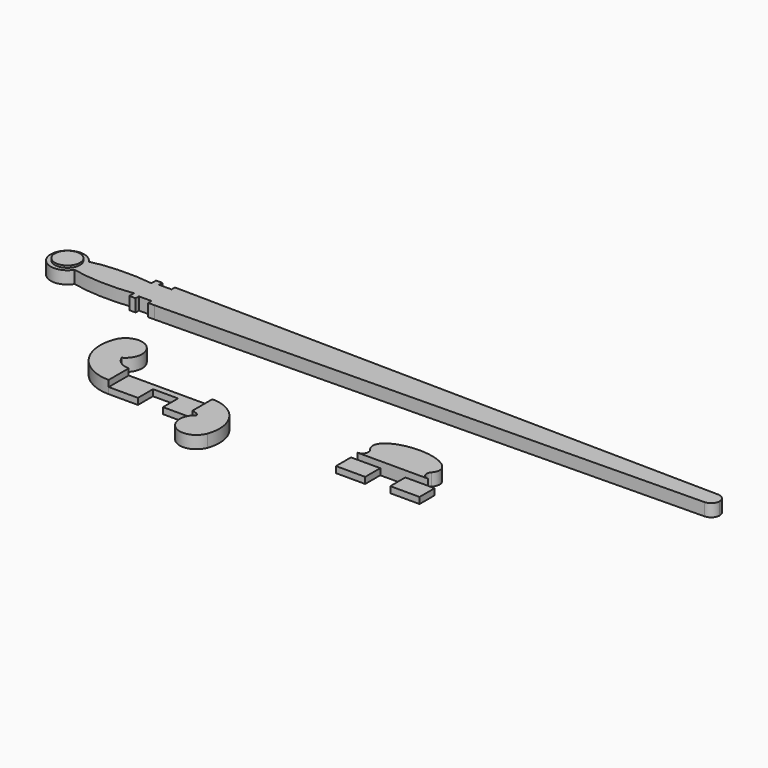
from build123d import *

# Parameters (mm, degrees)
F1_DEPTH      = 15
F0_W          = 35
F0_H          = 7.5
F2_DEPTH      = 7.5
F3_DEPTH      = 7.5
F4_DEPTH      = 17.5
F4_DEPTH_BACK = 2.5


# Not quite as in the source:
# - a feature names something its author has since deleted; it is built from what else it names


with BuildPart() as f1:
    # F0 (on Top) → F1 (new body)
    with BuildSketch(Plane.XY):
        with BuildLine():
            Line((90, 20), (90, 12.9903810568))
            add(Edge.make_bspline(
                [(90, -12.9903810568), (180, 0), (90, 12.9903810568)],
                knots=[2.0943951024, 2.0943951024, 2.0943951024, 4.1887902048, 4.1887902048, 4.1887902048], degree=2, weights=[1, 0.5, 1]))
            Line((90, -12.9903810568), (90, -20))
            Line((90, -20), (97.5, -20))
            Line((97.5, -20), (97.5, -15))
            Line((97.5, -15), (112.5, -15))
            Line((112.5, -15), (112.5, -20))
            Line((112.5, -20), (120, -20))
            Line((120, -20), (770.1538097556, -9.998817058))
            ThreePointArc((770.1538097556, -9.998817058), (760, 0), (770.1538097556, 9.998817058))
            Line((770.1538097556, 9.998817058), (120, 20))
            Line((120, 20), (112.5, 20))
            Line((112.5, 20), (112.5, 15))
            Line((112.5, 15), (97.5, 15))
            Line((97.5, 15), (97.5, 20))
            Line((97.5, 20), (90, 20))
        make_face()
        with BuildLine():
            add(Edge.make_bspline(
                [(90, -12.9903810568), (180, 0), (90, 12.9903810568)],
                knots=[2.0943951024, 2.0943951024, 2.0943951024, 4.1887902048, 4.1887902048, 4.1887902048], degree=2, weights=[1, 0.5, 1]))
            Line((90, 12.9903810568), (90, -12.9903810568))
        make_face()
        with BuildLine():
            ThreePointArc((17.0396451174, -10.4714131937), (19.2456865602, -5.4409143373), (20, 0))
            ThreePointArc((20, 0), (19.2456865602, 5.4409143373), (17.0396451174, 10.4714131937))
            add(Edge.make_bspline(
                [(17.0396451174, 10.4714131937), (14.3294049387, 9.7764683129), (12, 9)],
                knots=[5.5104529682, 5.5104529682, 5.5104529682, 5.6396841984, 5.6396841984, 5.6396841984], degree=2, weights=[1, 0.9979131374, 1]))
            ThreePointArc((12, 9), (14.2302494708, 4.7434164903), (15, 0))
            ThreePointArc((15, 0), (14.2302494708, -4.7434164903), (12, -9))
            add(Edge.make_bspline(
                [(12, -9), (14.3294049387, -9.7764683129), (17.0396451174, -10.4714131937)],
                knots=[0.6435011088, 0.6435011088, 0.6435011088, 0.7727323389, 0.7727323389, 0.7727323389], degree=2, weights=[1, 0.9979131374, 1]))
        make_face()
        with BuildLine():
            add(Edge.make_bspline(
                [(17.0396451174, 10.4714131937), (14.3294049387, 9.7764683129), (12, 9)],
                knots=[5.5104529682, 5.5104529682, 5.5104529682, 5.6396841984, 5.6396841984, 5.6396841984], degree=2, weights=[1, 0.9979131374, 1]))
            ThreePointArc((17.0396451174, 10.4714131937), (-20, 0), (17.0396451174, -10.4714131937))
            add(Edge.make_bspline(
                [(12, -9), (14.3294049387, -9.7764683129), (17.0396451174, -10.4714131937)],
                knots=[0.6435011088, 0.6435011088, 0.6435011088, 0.7727323389, 0.7727323389, 0.7727323389], degree=2, weights=[1, 0.9979131374, 1]))
            ThreePointArc((12, -9), (-15, 0), (12, 9))
        make_face()
        with BuildLine():
            ThreePointArc((17.0396451174, 10.4714131937), (19.2456865602, 5.4409143373), (20, 0))
            ThreePointArc((20, 0), (19.2456865602, -5.4409143373), (17.0396451174, -10.4714131937))
            add(Edge.make_bspline(
                [(17.0396451174, -10.4714131937), (49.6031402439, -18.8211655204), (90, -12.9903810568)],
                knots=[0.7727323389, 0.7727323389, 0.7727323389, 2.0943951024, 2.0943951024, 2.0943951024], degree=2, weights=[1, 0.7894822244, 1]))
            Line((90, -12.9903810568), (90, 12.9903810568))
            add(Edge.make_bspline(
                [(90, 12.9903810568), (49.6031402439, 18.8211655204), (17.0396451174, 10.4714131937)],
                knots=[4.1887902048, 4.1887902048, 4.1887902048, 5.5104529682, 5.5104529682, 5.5104529682], degree=2, weights=[1, 0.7894822244, 1]))
        make_face()
        with BuildLine():
            ThreePointArc((780, 0), (777.1252402611, 7.0164771233), (770.1538097556, 9.998817058))
            ThreePointArc((770.1538097556, 9.998817058), (760, 0), (770.1538097556, -9.998817058))
            ThreePointArc((770.1538097556, -9.998817058), (777.1252402611, -7.0164771233), (780, 0))
        make_face()
    extrude(amount=F1_DEPTH)


with BuildPart() as f1b:
    # F0 (on Top) → F1, piece 2 (new body)
    with BuildSketch(Plane.XY):
        with BuildLine():
            Line((181.0074592861, -142.1465528079), (181.0074592861, -134.6465528079))
            ThreePointArc((181.0074592861, -134.6465528079), (169.7383256758, -131.1694650111), (162.3875687612, -121.9472155752))
            ThreePointArc((162.3875687612, -121.9472155752), (165.8599218849, -89.2243569553), (134.0228282468, -97.5455456416))
            ThreePointArc((134.0228282468, -97.5455456416), (140.0498570717, -143.3253746254), (181.0074592861, -164.6465528079))
            Line((181.0074592861, -164.6465528079), (181.0074592861, -149.6465528079))
            Line((181.0074592861, -149.6465528079), (181.0074592861, -142.1465528079))
        make_face()
    extrude(amount=F1_DEPTH)



with BuildPart() as f1c:
    # F0 (on Top) → F1, piece 3 (new body)
    with BuildSketch(Plane.XY):
        with BuildLine():
            ThreePointArc((320.9443956695, -191.6824088992), (315.8214211684, -152.769554263), (281.0074592861, -134.6465528079))
            Line((281.0074592861, -134.6465528079), (281.0074592861, -142.1465528079))
            Line((281.0074592861, -142.1465528079), (281.0074592861, -149.6465528079))
            Line((281.0074592861, -149.6465528079), (281.0074592861, -164.6465528079))
            ThreePointArc((281.0074592861, -164.6465528079), (286.0735380817, -165.7191801598), (290.2701745279, -168.7529775059))
            ThreePointArc((290.2701745279, -168.7529775059), (290.1760382458, -200.8610955765), (320.9443956695, -191.6824088992))
        make_face()
    extrude(amount=F1_DEPTH)


with BuildPart() as f1d:
    # F0 (on Top) → F1, piece 4 (new body)
    with BuildSketch(Plane.XY):
        with BuildLine():
            add(Edge.make_bspline(
                [(527.8355032662, -126.8409866095), (531.1499030026, -124.7711446375), (533.2711188339, -122.3409866095)],
                knots=[5.6080537742, 5.6080537742, 5.6080537742, 5.8716684611, 5.8716684611, 5.8716684611], degree=2, weights=[1, 0.991325981, 1]))
            add(Edge.make_bspline(
                [(533.2711188339, -122.3409866095), (557.7115225403, -94.3409866095), (496.6105132742, -94.3409866095), (435.5095040081, -94.3409866095), (459.9499077146, -122.3409866095)],
                knots=[5.8716684611, 5.8716684611, 5.8716684611, 7.853981634, 7.853981634, 9.8362948068, 9.8362948068, 9.8362948068], degree=2, weights=[1, 0.5477225575, 1, 0.5477225575, 1]))
            add(Edge.make_bspline(
                [(459.9499077146, -122.3409866095), (462.0711235458, -124.7711446375), (465.3855232822, -126.8409866095)],
                knots=[3.5531094997, 3.5531094997, 3.5531094997, 3.8167241865, 3.8167241865, 3.8167241865], degree=2, weights=[1, 0.991325981, 1]))
            Line((465.3855232822, -126.8409866095), (527.8355032662, -126.8409866095))
        make_face()
        with BuildLine():
            add(Edge.make_bspline(
                [(465.3855232822, -126.8409866095), (477.3951348176, -134.3409866095), (496.6105132742, -134.3409866095)],
                knots=[3.8167241865, 3.8167241865, 3.8167241865, 4.7123889804, 4.7123889804, 4.7123889804], degree=2, weights=[1, 0.9013878189, 1]))
            add(Edge.make_bspline(
                [(496.6105132742, -134.3409866095), (515.8258917308, -134.3409866095), (527.8355032662, -126.8409866095)],
                knots=[4.7123889804, 4.7123889804, 4.7123889804, 5.6080537742, 5.6080537742, 5.6080537742], degree=2, weights=[1, 0.9013878189, 1]))
            Line((527.8355032662, -126.8409866095), (465.3855232822, -126.8409866095))
        make_face()
        with BuildLine():
            Line((454.4959551719, -134.3409866095), (481.6105132742, -134.3409866095))
            Line((481.6105132742, -134.3409866095), (496.6105132742, -134.3409866095))
            add(Edge.make_bspline(
                [(465.3855232822, -126.8409866095), (477.3951348176, -134.3409866095), (496.6105132742, -134.3409866095)],
                knots=[3.8167241865, 3.8167241865, 3.8167241865, 4.7123889804, 4.7123889804, 4.7123889804], degree=2, weights=[1, 0.9013878189, 1]))
            add(Edge.make_bspline(
                [(459.9499077146, -122.3409866095), (462.0711235458, -124.7711446375), (465.3855232822, -126.8409866095)],
                knots=[3.5531094997, 3.5531094997, 3.5531094997, 3.8167241865, 3.8167241865, 3.8167241865], degree=2, weights=[1, 0.991325981, 1]))
            ThreePointArc((459.9499077146, -122.3409866095), (461.0865848523, -130.097001804), (454.4959551719, -134.3409866095))
        make_face()
        with BuildLine():
            Line((496.6105132742, -134.3409866095), (511.6105132742, -134.3409866095))
            Line((511.6105132742, -134.3409866095), (538.7250713765, -134.3409866095))
            ThreePointArc((538.7250713765, -134.3409866095), (532.1344416961, -130.097001804), (533.2711188339, -122.3409866095))
            add(Edge.make_bspline(
                [(527.8355032662, -126.8409866095), (531.1499030026, -124.7711446375), (533.2711188339, -122.3409866095)],
                knots=[5.6080537742, 5.6080537742, 5.6080537742, 5.8716684611, 5.8716684611, 5.8716684611], degree=2, weights=[1, 0.991325981, 1]))
            add(Edge.make_bspline(
                [(496.6105132742, -134.3409866095), (515.8258917308, -134.3409866095), (527.8355032662, -126.8409866095)],
                knots=[4.7123889804, 4.7123889804, 4.7123889804, 5.6080537742, 5.6080537742, 5.6080537742], degree=2, weights=[1, 0.9013878189, 1]))
        make_face()
    extrude(amount=F1_DEPTH)

    # F0 (on Top) → F2 (join)
    with BuildSketch(Plane.XY):
        Polygon((511.6105132742, -141.8409866095), (546.6105132742, -141.8409866095), (546.6105132742, -134.3409866095), (538.7250713765, -134.3409866095), (511.6105132742, -134.3409866095), align=None)
        Polygon((446.6105132742, -141.8409866095), (481.6105132742, -141.8409866095), (481.6105132742, -134.3409866095), (454.4959551719, -134.3409866095), (446.6105132742, -134.3409866095), align=None)
        with Locations((529.1105132742, -153.0909866095)):
            Rectangle(F0_W, F0_H)
        with Locations((529.1105132742, -145.5909866095)):
            Rectangle(F0_W, F0_H)
        with Locations((464.1105132742, -153.0909866095)):
            Rectangle(F0_W, F0_H)
        with Locations((464.1105132742, -145.5909866095)):
            Rectangle(F0_W, F0_H)
    extrude(amount=F2_DEPTH)


with BuildPart() as f1b_1:
    add(f1b.part)

    add(f1c.part)  # F3 merges F1c
    # F0 (on Top) → F3 (join)
    with BuildSketch(Plane.XY):
        Polygon((281.0074592861, -134.6465528079), (181.0074592861, -134.6465528079), (181.0074592861, -142.1465528079), (216.0074592861, -142.1465528079), (246.0074592861, -142.1465528079), (281.0074592861, -142.1465528079), align=None)
        Polygon((216.0074592861, -142.1465528079), (181.0074592861, -142.1465528079), (181.0074592861, -149.6465528079), (181.0074592861, -164.6465528079), (216.0074592861, -164.6465528079), (216.0074592861, -157.1465528079), align=None)
        Polygon((281.0074592861, -149.6465528079), (281.0074592861, -142.1465528079), (246.0074592861, -142.1465528079), (246.0074592861, -157.1465528079), (246.0074592861, -164.6465528079), (281.0074592861, -164.6465528079), align=None)
    extrude(amount=F3_DEPTH)


with BuildPart() as f4:
    # F0 (on Top) → F4 (new body, two sides)
    with BuildSketch(Plane.XY) as f4_sk:
        with BuildLine():
            add(Edge.make_bspline(
                [(12, 9), (0, 5), (0, 0)],
                knots=[5.6396841984, 5.6396841984, 5.6396841984, 6.2831853072, 6.2831853072, 6.2831853072], degree=2, weights=[1, 0.9486832981, 1]))
            ThreePointArc((12, 9), (-15, 0), (12, -9))
            add(Edge.make_bspline(
                [(0, 0), (0, -5), (12, -9)],
                knots=[0, 0, 0, 0.6435011088, 0.6435011088, 0.6435011088], degree=2, weights=[1, 0.9486832981, 1]))
        make_face()
        with BuildLine():
            ThreePointArc((15, 0), (14.2302494708, 4.7434164903), (12, 9))
            add(Edge.make_bspline(
                [(12, 9), (0, 5), (0, 0)],
                knots=[5.6396841984, 5.6396841984, 5.6396841984, 6.2831853072, 6.2831853072, 6.2831853072], degree=2, weights=[1, 0.9486832981, 1]))
            add(Edge.make_bspline(
                [(0, 0), (0, -5), (12, -9)],
                knots=[0, 0, 0, 0.6435011088, 0.6435011088, 0.6435011088], degree=2, weights=[1, 0.9486832981, 1]))
            ThreePointArc((12, -9), (14.2302494708, -4.7434164903), (15, 0))
        make_face()
    extrude(amount=F4_DEPTH)
    extrude(f4_sk.sketch, amount=-F4_DEPTH_BACK)


solid = Compound([f1.part, f1d.part, f1b_1.part, f4.part])
